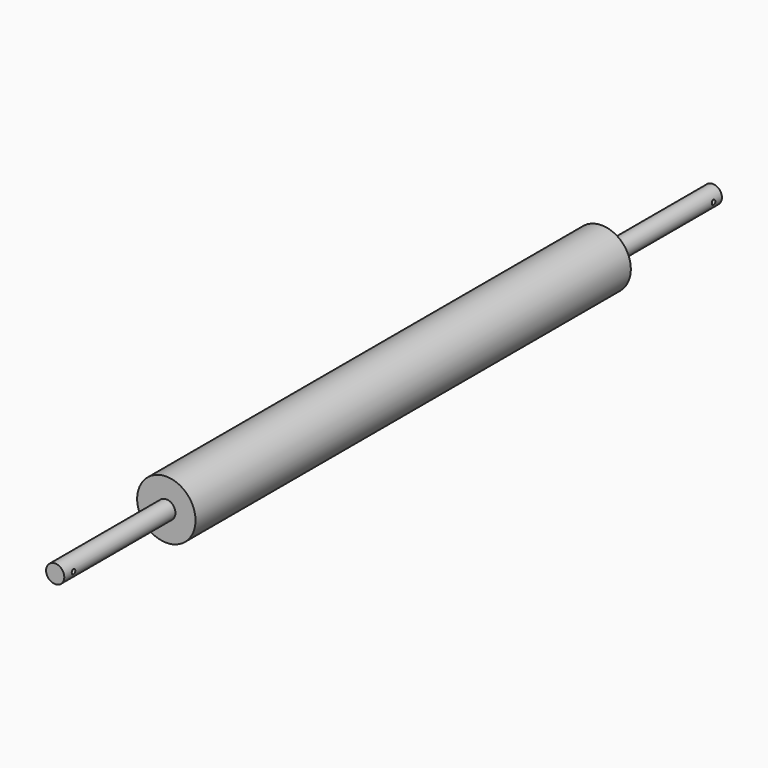
from build123d import *

# Parameters (mm, degrees)
F0_R     = 32
F0_R_2   = 10
F1_DEPTH = 596.9
F2_DEPTH = 152.4
F3_R     = 10
F4_DEPTH = 152.4
F5_R     = 2.5
F5_R_2   = 2.5019
F6_DEPTH = 63.5


# Not quite as in the source:
# - a feature names something its author has since deleted; it is built from what else it names


with BuildPart() as f1:
    # F0 (on Front) → F1 (new body)
    with BuildSketch(Plane.XZ):
        Circle(F0_R)
        Circle(F0_R_2, mode=Mode.SUBTRACT)
        Circle(F0_R_2)
    extrude(amount=-F1_DEPTH)

    # F0 (on Front) → F2 (join)
    with BuildSketch(Plane.XZ):
        Circle(F0_R_2)
    extrude(amount=F2_DEPTH)

    # F3 (on face) → F4 (join)
    with BuildSketch(Plane(origin=(0, 596.9, 0), x_dir=(-1, 0, 0), z_dir=(0, 1, 0))):
        Circle(F3_R)
    extrude(amount=F4_DEPTH)

    # F5 (on Right) → F6 (cut, symmetric)
    with BuildSketch(Plane.YZ):
        with Locations((-139.7, 0)):
            Circle(F5_R)
        with Locations((737.87, 0)):
            Circle(F5_R_2)
    extrude(amount=F6_DEPTH, both=True, mode=Mode.SUBTRACT)


solid = f1.part
